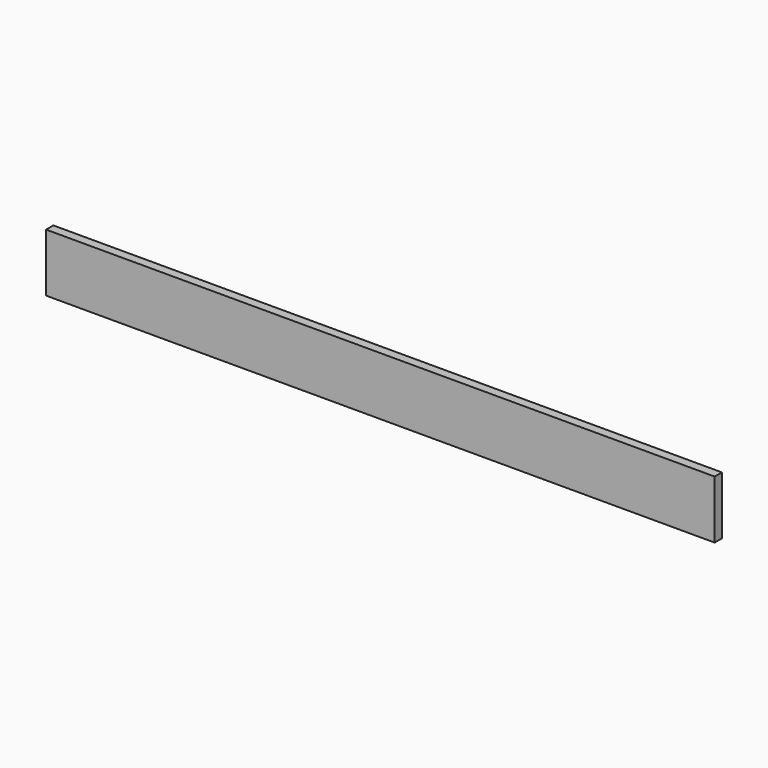
from build123d import *

# Parameters (mm, degrees)
F0_W     = 1168.4
F0_H     = 15.875
F1_DEPTH = 101.6


# Not quite as in the source:
# - a feature names something its author has since deleted; it is built from what else it names


with BuildPart() as f1:
    # F0 (on Top) → F1 (new body)
    with BuildSketch(Plane.XY):
        with Locations((584.2, 7.9375)):
            Rectangle(F0_W, F0_H)
    extrude(amount=F1_DEPTH)


solid = f1.part
